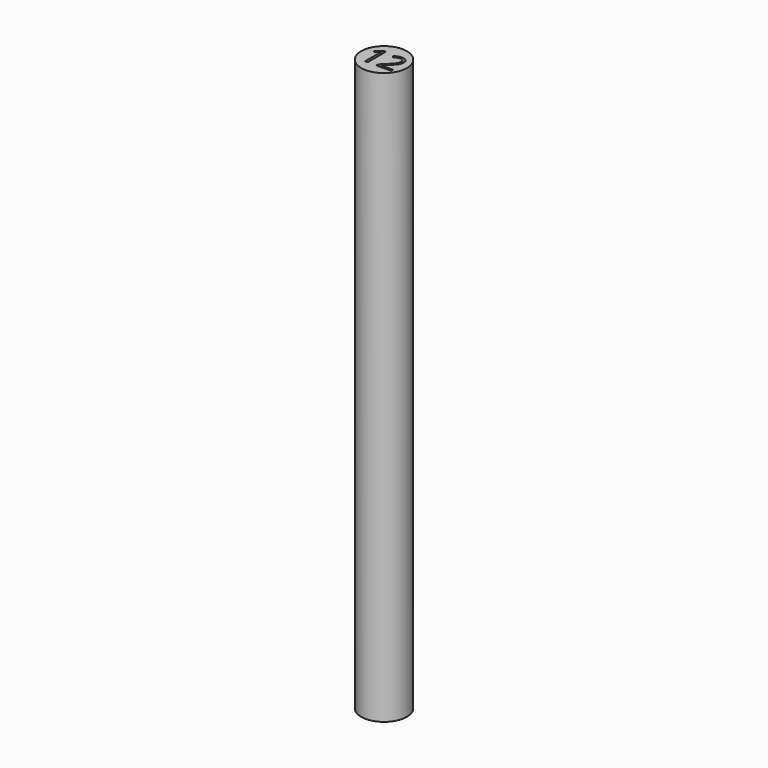
from build123d import *

# Parameters (mm, degrees)
F0_R         = 6
F1_DEPTH     = 150
F2_TEXT_SIZE = 8.3333333333
F3_DEPTH     = 1
F4_TEXT_SIZE = 8.3333333333
F5_DEPTH     = 1


# Not quite as in the source:
# - Text() gives the source's letters only with a copy of the font that has no kerning and outlines rounded to 1/6400 em; it was checked with that copy


with BuildPart() as f1:
    # F0 (on Top) → F1 (new body)
    with BuildSketch(Plane.XY):
        Circle(F0_R)
    extrude(amount=F1_DEPTH)

    # F2 (on face) → F3 (cut)
    with BuildSketch(Plane(origin=(0, 0, 0), x_dir=(1, 0, 0), z_dir=(0, 0, -1))):
        with Locations((-4.8111979167, -3)):
            Text('12', F2_TEXT_SIZE, font='Open Sans', text_align=(TextAlign.LEFT, TextAlign.BOTTOM))
    extrude(amount=-F3_DEPTH, mode=Mode.SUBTRACT)

    # F4 (on face) → F5 (cut)
    with BuildSketch(Plane.XY.offset(150)):
        with Locations((-4.8111979167, -3)):
            Text('12', F4_TEXT_SIZE, font='Open Sans', text_align=(TextAlign.LEFT, TextAlign.BOTTOM))
    extrude(amount=-F5_DEPTH, mode=Mode.SUBTRACT)


solid = f1.part
